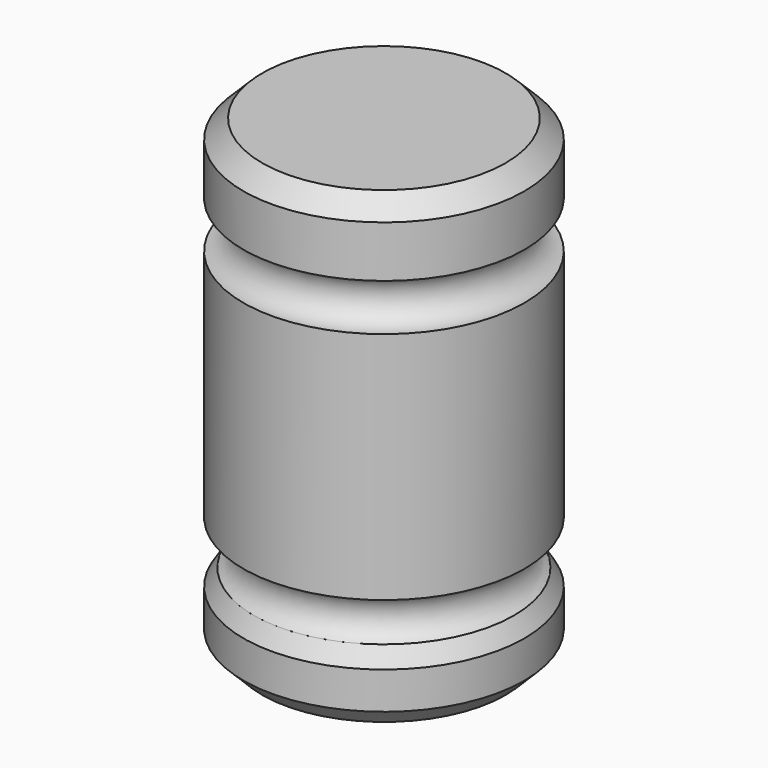
from build123d import *


# Not quite as in the source:
# - a fillet or chamfer that OpenCascade refuses, or shapes differently, is made with other operations: its cross-section is extruded or revolved along the edge and cut away or added


with BuildPart() as f1:
    # F0 (on Front) → F1 (revolve)
    with BuildSketch(Plane.XZ):
        with BuildLine():
            Line((-38.1, 0), (0, 0))
            Line((0, 0), (0, 19.05))
            ThreePointArc((0, 19.05), (-6.35, 25.4), (0, 31.75))
            Line((0, 31.75), (0, 95.25))
            ThreePointArc((0, 95.25), (-6.35, 101.6), (0, 107.95))
            Line((0, 107.95), (0, 127))
            Line((0, 127), (-38.1, 127))
            Line((-38.1, 127), (-38.1, 0))
        make_face()
    revolve(axis=Axis((-38.1, 0, 63.5), (0, 0, 1)))

    # F2: chamfer of 5.08 on 4 edges, made by hand

    # F2_s1 → F2_t2 (revolve, cut)
    with BuildSketch(Plane.XZ):
        Polygon((0, 121.92), (-5.08, 127), (0, 127), align=None)
    revolve(axis=Axis((-38.1, 0, 127), (0, 0, 1)), mode=Mode.SUBTRACT)

    # F2_s3 → F2_t4 (revolve, cut)
    with BuildSketch(Plane.XZ):
        Polygon((-5.08, 0), (0, 5.08), (0, 0), align=None)
    revolve(axis=Axis((-38.1, 0, 0), (0, 0, 1)), mode=Mode.SUBTRACT)

    # F2_s5 → F2_t6 (revolve, cut)
    with BuildSketch(Plane.XZ):
        with BuildLine():
            Line((0, 15.1609326597), (-2.8222222222, 19.7116292554))
            ThreePointArc((-2.8222222222, 19.7116292554), (-1.5219513398, 19.2350860412), (0, 19.05))
            Line((0, 19.05), (0, 15.1609326597))
        make_face()
    revolve(axis=Axis((-38.1, 0, 19.05), (0, 0, 1)), mode=Mode.SUBTRACT)


solid = f1.part
